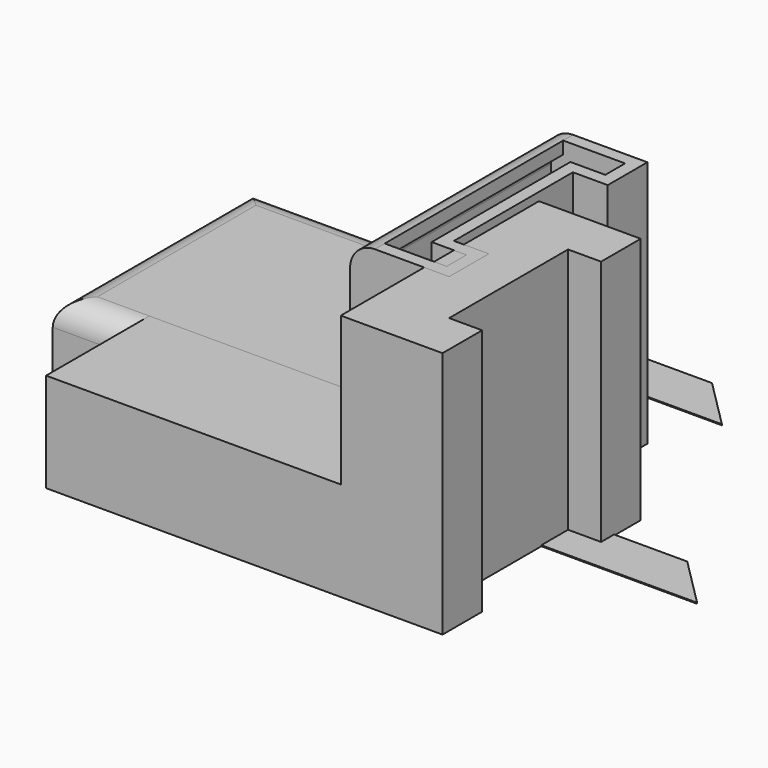
from build123d import *

# Parameters (mm, degrees)
F1_DEPTH     = 0.2
F2_W         = 60
F2_H         = 50
F3_DEPTH     = 20
F4_DEPTH     = 50
F5_W         = 59.4666637367
F5_H         = 50
F6_DEPTH     = 20
F7_DEPTH     = 50
F8_R         = 5
F9_T         = 2.5
F9_T3_DEPTH  = 45
F9_T5_DEPTH  = 55
F9_T8_ANGLE  = 90.000000001
F9_T10_ANGLE = 90.000000001


# Not quite as in the source:
# - a shell that OpenCascade refuses in one call is made with other operations: the cavity is built on its own and cut out


with BuildPart() as f1:
    # F0 (on Top) → F1 (new body)
    with BuildSketch(Plane.XY):
        Polygon((23.8681607499, 43.2712367737), (13.8681607499, 53.2712367737), (-1.1318392501, 53.2712367737), (-1.1318392501, -6.7287632263), (58.8681607499, -6.7287632263), (48.8681607499, 3.2712367737), (8.8681607499, 3.2712367737), (8.8681607499, 43.2712367737), align=None)
    extrude(amount=F1_DEPTH)


with BuildPart() as f3:
    # F2 (on Top) → F3 (new body)
    with BuildSketch(Plane.XY):
        with Locations((-31.3888411792, 6.0425736521)):
            Rectangle(F2_W, F2_H)
    extrude(amount=F3_DEPTH)

    # F2 (on Top) → F4 (join)
    with BuildSketch(Plane.XY):
        Polygon((-1.3888411792, 31.0425736521), (-1.3888411792, -18.9574263479), (18.6111588208, -18.9574263479), (18.6111588208, -8.9574263479), (11.5741182365, -8.9574263479), (11.5741182365, 21.0425736521), (18.6111588208, 21.0425736521), (18.6111588208, 31.0425736521), align=None)
    extrude(amount=F4_DEPTH)

    # F8
    f8_edges = [f3.edges().sort_by_distance(p)[0] for p in [
        (-1.388841, 6.042574, 50),
        (-61.388841, 6.042574, 20),
        (-31.388841, -18.957426, 20),
        (-31.388841, 31.042574, 20),
    ]]
    fillet(f8_edges, radius=F8_R)

    # F9: shell of thickness 2.5, made by hand


with BuildPart() as f6:
    # F5 (on Top) → F6 (new body)
    with BuildSketch(Plane.XY):
        with Locations((-16.1652588892, -15)):
            Rectangle(F5_W, F5_H)
    extrude(amount=F6_DEPTH)

    # F5 (on Top) → F7 (join)
    with BuildSketch(Plane.XY):
        Polygon((13.5680729791, 10), (13.5680729791, -40), (34.1014092424, -40), (34.1014092424, -30), (27.4347461201, -30), (27.4347461201, 0), (34.1014092424, 0), (34.1014092424, 10), align=None)
    extrude(amount=F7_DEPTH)


with BuildPart() as f9_core1:
    # F9_t2: copy of F3
    add(f3.part)

    # the walls: a layer under each face that stays
    f9_faces = [f9_core1.faces().sort_by_distance(p)[0] for p in [
        (-61.3888411792, 6.0425736521, 7.5),
        (5.2778254875, 31.0425736521, 41.6666666667),
        (-59.9243750851, 6.0425736521, 18.5355339059),
        (-21.3888411792, 6.0425736521, 0),
        (-48.0555078458, -18.9574263479, 8.3333333333),
        (-31.3888411792, 29.578107558, 18.5355339059),
        (-1.3888411792, 6.0425736521, 30),
        (18.6111588208, 26.0425736521, 25),
        (0.0756249149, 6.0425736521, 48.5355339059),
        (-28.8888411792, 6.0425736521, 20),
        (-31.3888411792, -17.4929602538, 18.5355339059),
        (18.6111588208, -13.9574263479, 25),
        (15.0926385287, -8.9574263479, 25),
        (11.5741182365, 6.0425736521, 25),
        (15.0926385287, 21.0425736521, 25),
    ]]
    thicken(f9_faces, amount=-F9_T, mode=Mode.SUBTRACT)

    # F9_s4 → F9_t3 (cut)
    with BuildSketch(Plane.XZ.offset(-28.5425736521)):
        Polygon((-1.4138411792, 20.025), (1.1111588208, 20), (1.1111588208, 17.5), (-1.3888411792, 17.5), align=None)
    extrude(amount=F9_T3_DEPTH, mode=Mode.SUBTRACT)

    # F9_s6 → F9_t5 (cut)
    with BuildSketch(Plane.XY.offset(-2.5)):
        Polygon((11.5991182365, -8.9324263479), (11.5741182365, -11.4574263479), (9.0741182365, -11.4574263479), (9.0741182365, -8.9574263479), align=None)
        Polygon((11.5991182365, 21.0175736521), (9.0741182365, 21.0425736521), (9.0741182365, 23.5425736521), (11.5741182365, 23.5425736521), align=None)
    extrude(amount=F9_T5_DEPTH, mode=Mode.SUBTRACT)

    # F9_s7 → F9_t8 (revolve, cut)
    with BuildSketch(Plane.XZ.offset(-26.0425736521)):
        Polygon((-1.4138411792, 20.025), (-1.3888411792, 17.5), (1.1111588208, 17.5), (1.1111588208, 20), align=None)
    revolve(axis=Axis((-1.3888411792, 26.0425736521, 15), (-1, 0, 0)), revolution_arc=F9_T8_ANGLE, mode=Mode.SUBTRACT)

    # F9_s9 → F9_t10 (revolve, cut)
    with BuildSketch(Plane.XZ.offset(13.9574263479)):
        Polygon((-1.4138411792, 20.025), (1.1111588208, 20), (1.1111588208, 17.5), (-1.3888411792, 17.5), align=None)
    revolve(axis=Axis((-1.3888411792, -13.9574263479, 15), (1, 0, 0)), revolution_arc=F9_T10_ANGLE, mode=Mode.SUBTRACT)


with BuildPart() as f3_1:
    add(f3.part)

    # what is left inside the walls is the cavity
    f9_cavity = [f9_core1.part.solids().sort_by_distance(p)[0] for p in [
        (-21.388841, -1.457426, 2.525),
    ]]
    add(f9_cavity, mode=Mode.SUBTRACT)


solid = Compound([f1.part, f6.part, f3_1.part])
